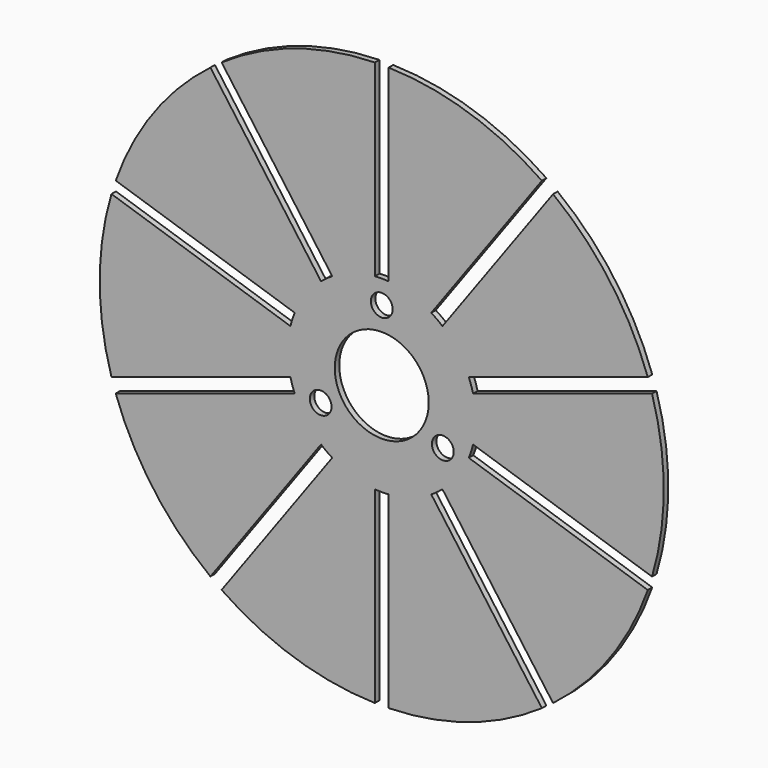
from build123d import *

# Parameters (mm, degrees)
F0_R            = 38.1
F0_R_2          = 6.35
F1_DEPTH        = 0.762
F3_DEPTH        = 0.763
F3_COPIES_COUNT = 10
F5_D            = 2.9464


# Not quite as in the source:
# - a pattern or mirror of a feature is missing from the dataset's text; its kind, count and spacing are read off the source's solid


with BuildPart() as f1:
    # F0 (on Front) → F1 (new body)
    with BuildSketch(Plane.XZ):
        Circle(F0_R)
        Circle(F0_R_2, mode=Mode.SUBTRACT)
    extrude(amount=F1_DEPTH)

    # F2 (on face) → F3 (cut, through all)
    with BuildSketch(Plane.XZ.offset(0.762)):
        with BuildLine():
            Line((-0.9345413193, 38.0885367601), (-0.9345413193, 12.6655687801))
            ThreePointArc((-0.9345413193, 12.6655687801), (0, 12.7), (0.9345413193, 12.6655687801))
            Line((0.9345413193, 12.6655687801), (0.9345413193, 38.0885367601))
            ThreePointArc((0.9345413193, 38.0885367601), (0, 38.1), (-0.9345413193, 38.0885367601))
        make_face()
    f3 = extrude(amount=-F3_DEPTH, mode=Mode.SUBTRACT)

    # F3_copies: F3 ×10 about axis
    f3_copies_axis = Axis((0, 0, 0), (0, 1, 0))
    for i in range(1, F3_COPIES_COUNT):
        add(f3.rotate(f3_copies_axis, i * 360 / F3_COPIES_COUNT), mode=Mode.SUBTRACT)

    # F5 (through all)
    with Locations(Plane.XZ.offset(0.762)):
        with Locations((0, 9.525), (-8.248891971, -4.7625), (8.248891971, -4.7625)):
            Hole(F5_D / 2)


solid = f1.part
